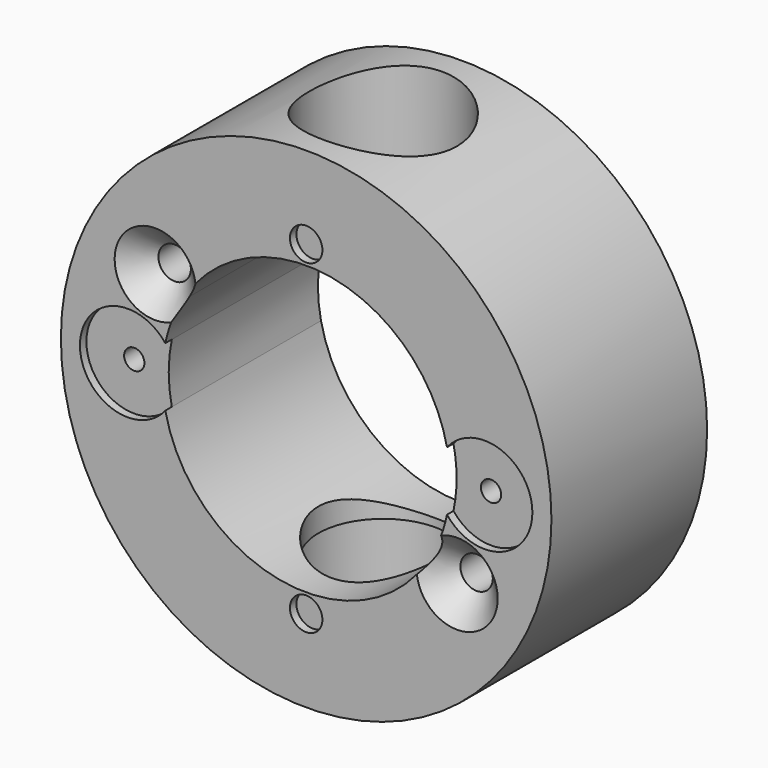
from build123d import *

# Parameters (mm, degrees)
F0_R          = 30.25
F0_R_2        = 2
F1_DEPTH      = 24
F0_R_3        = 1.25
F2_DEPTH      = 23
F5_R          = 9.125
F5_R_2        = 8
F6_DEPTH      = 25
F7_DEPTH      = 60
F7_DEPTH_BACK = 30
F8_START      = -37.5
F8_DEPTH      = 45.7


# Not quite as in the source:
# - a fillet or chamfer that OpenCascade refuses, or shapes differently, is made with other operations: its cross-section is extruded or revolved along the edge and cut away or added


with BuildPart() as f1:
    # F0 (on Front) → F1 (new body)
    with BuildSketch(Plane.XZ):
        Circle(F0_R)
        with Locations((0, -20.07)):
            Circle(F0_R_2, mode=Mode.SUBTRACT)
        with Locations((18.6195461814, -10.75)):
            Circle(F0_R_2, mode=Mode.SUBTRACT)
        with BuildLine():
            ThreePointArc((-16.6195461814, 10.75), (-16.6876945288, 10.2323619098), (-16.8874953738, 9.75))
            ThreePointArc((-16.8874953738, 9.75), (-20.5513978339, 11.2676380902), (-16.6195461814, 10.75))
        make_face(mode=Mode.SUBTRACT)
        with BuildLine():
            ThreePointArc((8.875, 15.3719509172), (14.3703479176, 10.4190019065), (17.369375, 3.6561334917))
            ThreePointArc((17.369375, 3.6561334917), (23.9351114309, 5.5736293158), (27.9, 0))
            ThreePointArc((27.9, 0), (23.9351114309, -5.5736293158), (17.369375, -3.6561334917))
            ThreePointArc((17.369375, -3.6561334917), (0, -17.75), (-17.369375, -3.6561334917))
            ThreePointArc((-17.369375, -3.6561334917), (-27.9, 0), (-17.369375, 3.6561334917))
            ThreePointArc((-17.369375, 3.6561334917), (-16.5773263107, 6.3446632999), (-15.3719509172, 8.875))
            ThreePointArc((-15.3719509172, 8.875), (-4.5940380506, 17.1451834166), (8.875, 15.3719509172))
        make_face(mode=Mode.SUBTRACT)
        with Locations((0, 20.07)):
            Circle(F0_R_2, mode=Mode.SUBTRACT)
    extrude(amount=F1_DEPTH)

    # F0 (on Front) → F2 (join)
    with BuildSketch(Plane.XZ):
        with BuildLine():
            ThreePointArc((-17.369375, 3.6561334917), (-27.9, 0), (-17.369375, -3.6561334917))
            ThreePointArc((-17.369375, -3.6561334917), (-17.75, 0), (-17.369375, 3.6561334917))
        make_face()
        with Locations((-22, 0)):
            Circle(F0_R_3, mode=Mode.SUBTRACT)
        with Locations((0, 20.07)):
            Circle(F0_R_2)
        with BuildLine():
            ThreePointArc((17.369375, 3.6561334917), (17.6545873111, 1.8379463744), (17.75, 0))
            ThreePointArc((17.75, 0), (17.6545873111, -1.8379463744), (17.369375, -3.6561334917))
            ThreePointArc((17.369375, -3.6561334917), (23.9351114309, -5.5736293158), (27.9, 0))
            ThreePointArc((27.9, 0), (23.9351114309, 5.5736293158), (17.369375, 3.6561334917))
        make_face()
        with Locations((22, 0)):
            Circle(F0_R_3, mode=Mode.SUBTRACT)
        with Locations((0, -20.07)):
            Circle(F0_R_2)
    extrude(amount=F2_DEPTH)

    # F3: chamfer of 3 on 2 edges, made by hand

    # F3_s1 → F3_t2 (revolve, cut)
    with BuildSketch(Plane.XY.offset(10.75)):
        Polygon((-13.6195461814, -24), (-16.6195461814, -21), (-16.6195461814, -24), align=None)
    revolve(axis=Axis((-18.6195461814, -24, 10.75), (0, -1, 0)), mode=Mode.SUBTRACT)

    # F3_s3 → F3_t4 (revolve, cut)
    with BuildSketch(Plane.XY.offset(-10.75)):
        Polygon((23.6195461814, -24), (20.6195461814, -21), (20.6195461814, -24), align=None)
    revolve(axis=Axis((18.6195461814, -24, -10.75), (0, -1, 0)), mode=Mode.SUBTRACT)

    # F5 (on offset) → F6 (cut)
    with BuildSketch(Plane.XY.offset(18.75)):
        with Locations((0, -12.125)):
            Circle(F5_R)
        with Locations((0, -12.125)):
            Circle(F5_R_2, mode=Mode.SUBTRACT)
    extrude(amount=F6_DEPTH, mode=Mode.SUBTRACT)

    # F5 (on offset) → F7 (cut, two sides)
    with BuildSketch(Plane.XY.offset(18.75)) as f7_sk:
        with Locations((0, -12.125)):
            Circle(F5_R_2)
    extrude(amount=-F7_DEPTH, mode=Mode.SUBTRACT)
    extrude(f7_sk.sketch, amount=F7_DEPTH_BACK, mode=Mode.SUBTRACT)

    # F5 (on offset) → F8 (cut)
    with BuildSketch(Plane.XY.offset(18.75).offset(F8_START)):
        with Locations((0, -12.125)):
            Circle(F5_R)
        with Locations((0, -12.125)):
            Circle(F5_R_2, mode=Mode.SUBTRACT)
    extrude(amount=-F8_DEPTH, mode=Mode.SUBTRACT)


solid = f1.part
